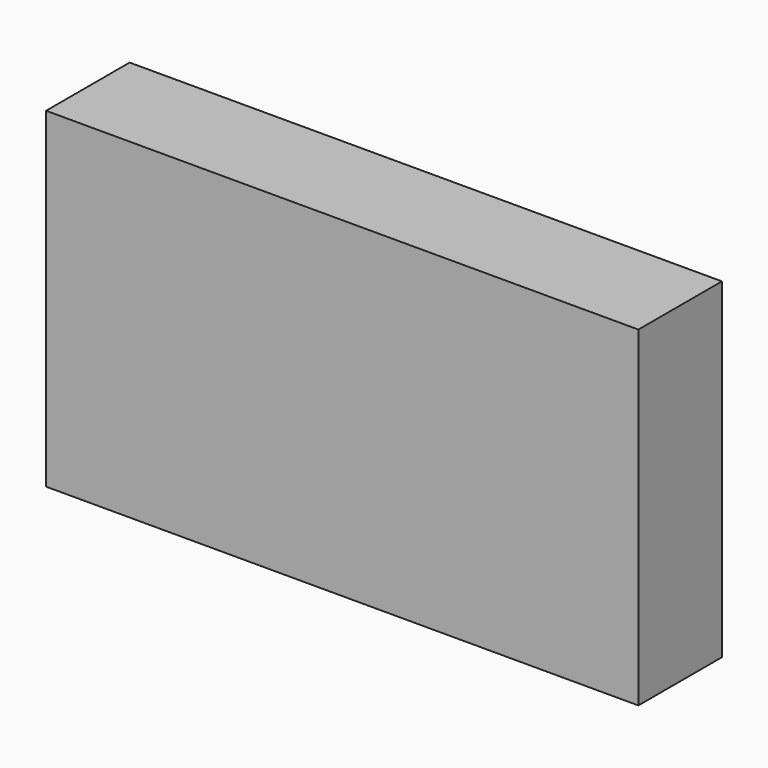
from build123d import *

# Parameters (mm, degrees)
F0_W     = 308.3597868681
F0_H     = 172.2804456949
F1_DEPTH = 54.356
F2_T     = -2.54


# Not quite as in the source:
# - the program builds the solid bodies; features that only make, move or delete a surface that nothing else refers to are left out


with BuildPart() as f1:
    # F0 (on Front) → F1 (new body)
    with BuildSketch(Plane.XZ):
        with Locations((-0.0235065818, 0.1487284899)):
            Rectangle(F0_W, F0_H)
    extrude(amount=F1_DEPTH)

    # F2
    f2_openings = [f1.faces().sort_by_distance(p)[0] for p in [
        (-0.023507, 0, 0.148728),
    ]]
    offset(amount=F2_T, openings=f2_openings)


solid = f1.part
